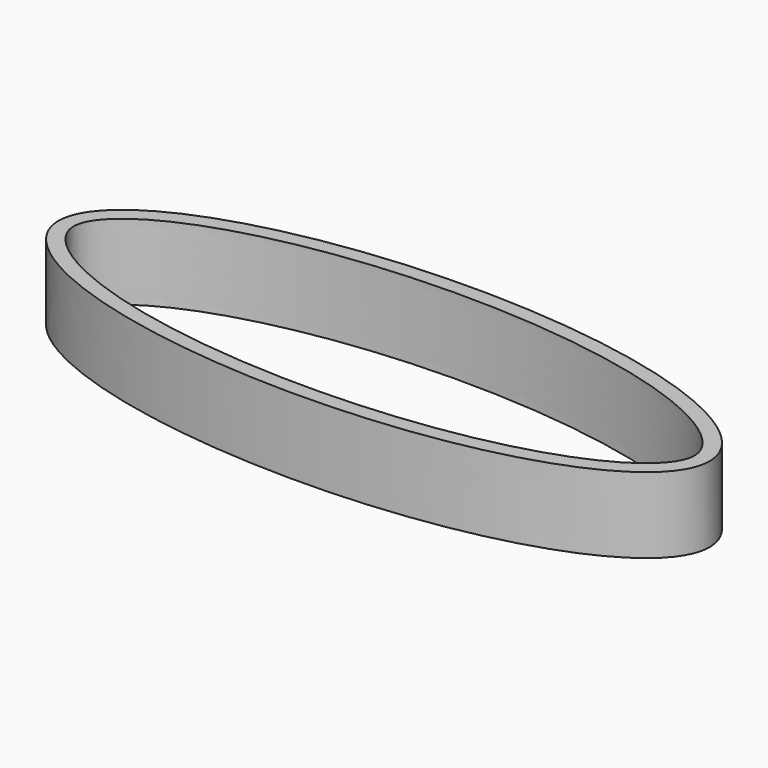
from build123d import *

# Parameters (mm, degrees)
F1_DEPTH = 5


# Not quite as in the source:
# - the dataset's text gives a spline's control points without its knots; the knots are read off the source's solid


with BuildPart() as f1:
    # F0 (on Top) → F1 (new body)
    with BuildSketch(Plane.XY):
        with BuildLine():
            add(Edge.make_bspline(
                [(23.1513766022, -1.5481652226), (23.1513766022, 11.4422158341), (-9.0986233978, 4.9470253058), (-41.3486233978, -1.5481652226), (-9.0986233978, -8.043355751), (23.1513766022, -14.5385462794), (23.1513766022, -1.5481652226)],
                knots=[0, 0, 0, 2.0943951024, 2.0943951024, 4.1887902048, 4.1887902048, 6.2831853072, 6.2831853072, 6.2831853072], degree=2, weights=[1, 0.5, 1, 0.5, 1, 0.5, 1]))
        make_face()
        with BuildLine():
            add(Edge.make_bspline(
                [(22.1513766022, -1.5481652226), (22.1513766022, -1.3957834945), (22.1096202891, -1.0910200383), (21.8997790745, -0.5881137177), (21.5054122724, -0.0330341465), (20.9071604219, 0.5537871587), (20.1014780687, 1.1503577264), (18.7558835435, 1.9345569489), (16.6265652431, 2.8406834353), (13.9883420294, 3.5980421453), (11.6157952827, 4.0943114302), (9.1190894258, 4.5058126497), (6.4713809105, 4.7858845153), (3.7357829569, 4.9278586626), (1.6513766022, 4.9638228348), (-0.4330297524, 4.9278586626), (-3.168627706, 4.7858845153), (-5.8163362213, 4.5058126497), (-8.3130420782, 4.0943114302), (-10.6855888249, 3.5980421453), (-13.3238120386, 2.8406834353), (-15.453130339, 1.9345569489), (-16.7987248643, 1.1503577264), (-17.6044072174, 0.5537871587), (-18.202659068, -0.0330341465), (-18.59702587, -0.5881137177), (-18.8068670846, -1.0910200383), (-18.8695015543, -1.5481652226), (-18.8068670846, -2.0053104069), (-18.59702587, -2.5082167276), (-18.202659068, -3.0632962987), (-17.6044072174, -3.650117604), (-16.7987248643, -4.2466881717), (-15.453130339, -5.0308873942), (-13.3238120386, -5.9370138806), (-10.6855888249, -6.6943725906), (-8.3130420782, -7.1906418755), (-5.8163362213, -7.602143095), (-3.168627706, -7.8822149606), (-0.4330297524, -8.0241891078), (1.6513766022, -8.06015328), (3.7357829569, -8.0241891078), (6.4713809105, -7.8822149606), (9.1190894258, -7.602143095), (11.6157952827, -7.1906418755), (13.9883420294, -6.6943725906), (16.6265652431, -5.9370138806), (18.7558835435, -5.0308873942), (20.1014780687, -4.2466881717), (20.9071604219, -3.650117604), (21.5054122724, -3.0632962987), (21.8997790745, -2.5082167276), (22.1096202891, -2.0053104069), (22.1513766022, -1.7005469507), (22.1513766022, -1.5481652226)],
                knots=[0, 0, 0, 0, 0.015625, 0.03125, 0.046875, 0.0625, 0.078125, 0.09375, 0.125, 0.15625, 0.171875, 0.1875, 0.21875, 0.234375, 0.25, 0.265625, 0.28125, 0.3125, 0.328125, 0.34375, 0.375, 0.40625, 0.421875, 0.4375, 0.453125, 0.46875, 0.484375, 0.5, 0.515625, 0.53125, 0.546875, 0.5625, 0.578125, 0.59375, 0.625, 0.65625, 0.671875, 0.6875, 0.71875, 0.734375, 0.75, 0.765625, 0.78125, 0.8125, 0.828125, 0.84375, 0.875, 0.90625, 0.921875, 0.9375, 0.953125, 0.96875, 0.984375, 1, 1, 1, 1], degree=3))
        make_face(mode=Mode.SUBTRACT)
    extrude(amount=F1_DEPTH)


solid = f1.part
